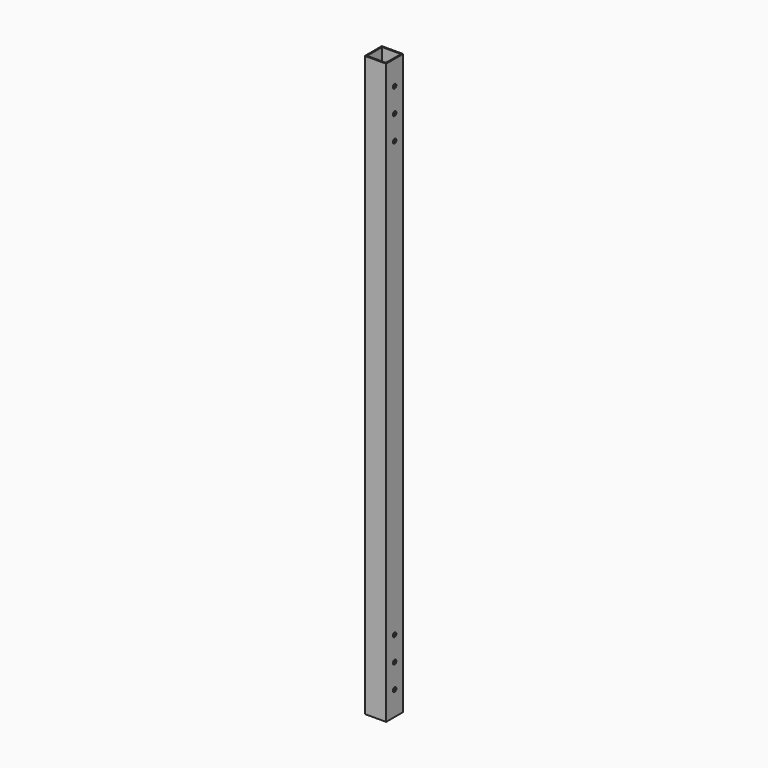
from build123d import *

# Parameters (mm, degrees)
F0_W     = 44
F0_H     = 44
F0_W_2   = 39
F0_H_2   = 39
F1_DEPTH = 1200
F3_D     = 8.8


# Not quite as in the source:
# - a feature names something its author has since deleted; it is built from what else it names


with BuildPart() as f1:
    # F0 (on Top) → F1 (new body)
    with BuildSketch(Plane.XY):
        Rectangle(F0_W, F0_H)
        Rectangle(F0_W_2, F0_H_2, mode=Mode.SUBTRACT)
    extrude(amount=F1_DEPTH)

    # F3 (through all)
    with Locations(Plane(origin=(-22, 0, 0), x_dir=(0, -1, 0), z_dir=(-1, 0, 0))):
        with Locations((0, 150), (0, 100), (0, 50), (0, 1050), (0, 1150), (0, 1100)):
            Hole(F3_D / 2)


solid = f1.part
